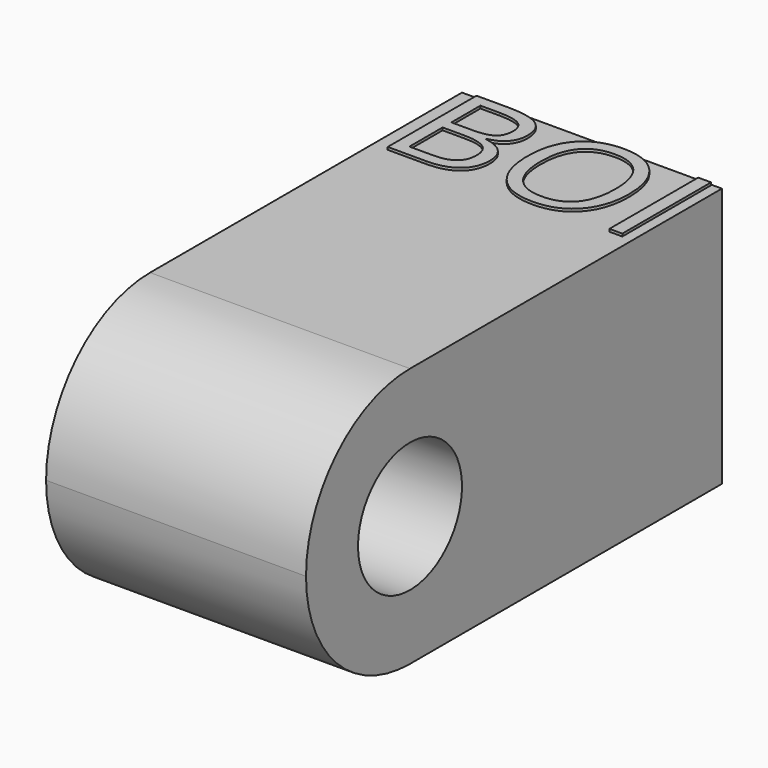
from build123d import *

# Parameters (mm, degrees)
F0_W         = 25.4
F0_H         = 25.4
F1_DEPTH     = 50.8
F3_R         = 12.69999
F2_R         = 6.35
F4_DEPTH     = 25.4
F5_TEXT_SIZE = 15.1854273704
F6_DEPTH     = 0.254


# Not quite as in the source:
# - a fillet or chamfer is up to 0.001 mm smaller than in the source, because OpenCascade refuses the exact size
# - Text() gives the source's letters only with a copy of the font that has no kerning and outlines rounded to 1/6400 em; it was checked with that copy


with BuildPart() as f1:
    # F0 (on Front) → F1 (new body)
    with BuildSketch(Plane.XZ):
        Rectangle(F0_W, F0_H)
    extrude(amount=F1_DEPTH)

    # F3 (radius 12.7 in the source; OpenCascade refuses exactly that, so slightly less here)
    f3_edges = [f1.edges().sort_by_distance(p)[0] for p in [
        (0, -50.8, 12.7),
        (0, -50.8, -12.7),
    ]]
    fillet(f3_edges, radius=F3_R)

    # F2 (on face) → F4 (cut)
    with BuildSketch(Plane(origin=(-12.7, 0, 0), x_dir=(0, -1, 0), z_dir=(-1, 0, 0))):
        with Locations((38.1, 0)):
            Circle(F2_R)
    extrude(amount=-F4_DEPTH, mode=Mode.SUBTRACT)

    # F5 (on face) → F6 (join)
    with BuildSketch(Plane.XY.offset(12.7)):
        with Locations((-12.7, -10.9335077067)):
            Text('BOI', F5_TEXT_SIZE, font='Open Sans', text_align=(TextAlign.LEFT, TextAlign.BOTTOM))
    extrude(amount=F6_DEPTH)


solid = f1.part
